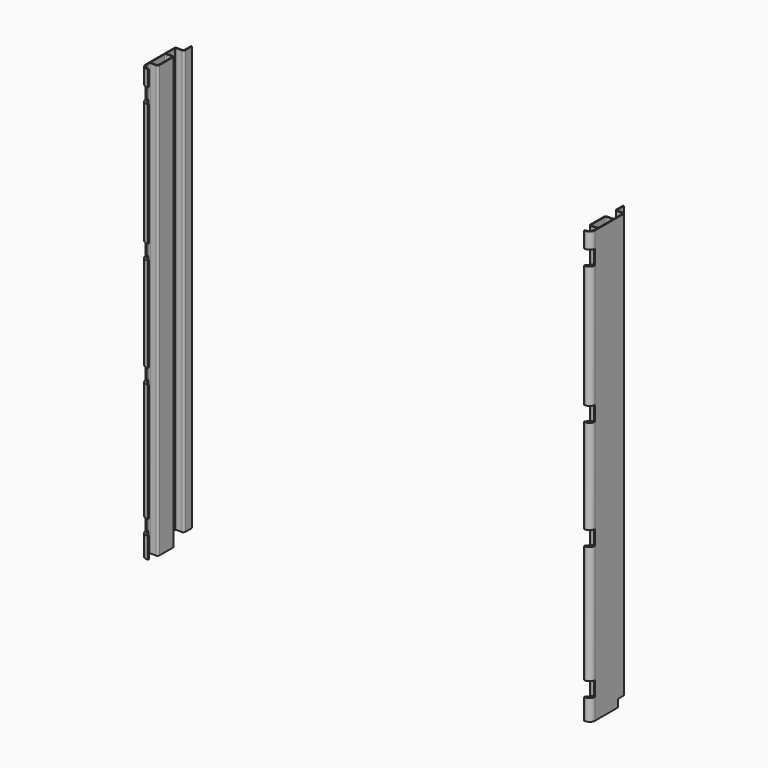
from build123d import *

# Parameters (mm, degrees)
F1_DEPTH  = 2337
F2_W      = 58.9122746438
F2_H      = 85
F2_W_2    = 42.5596956462
F2_W_3    = 40.1068006009
F2_W_4    = 37.0883546919
F2_H_2    = 41
F3_DEPTH  = 55
F5_DEPTH  = 2
F7_DEPTH  = 2
F9_DEPTH  = 2
F11_DEPTH = 2
F13_DEPTH = 2
F15_DEPTH = 2
F17_DEPTH = 2
F19_DEPTH = 2
F21_DEPTH = 2337


# Not quite as in the source:
# - a feature names something its author has since deleted; it is built from what else it names


with BuildPart() as f1:
    # F0 (on Top) → F1 (new body)
    with BuildSketch(Plane.XY):
        with BuildLine():
            Line((-45, 88.8779433221), (-45, 133.8779433221))
            Line((-45, 133.8779433221), (-50, 133.8779433221))
            Line((-50, 133.8779433221), (-50, 88.8779433221))
            ThreePointArc((-50, 88.8779433221), (-47.0710678119, 81.8068755102), (-40, 78.8779433221))
            Line((-40, 78.8779433221), (-10, 78.8779433221))
            ThreePointArc((-10, 78.8779433221), (-6.4644660941, 77.413477228), (-5, 73.8779433221))
            Line((-5, 73.8779433221), (-5, 19.8779433221))
            ThreePointArc((-5, 19.8779433221), (-6.4644660941, 16.3424094161), (-10, 14.8779433221))
            Line((-10, 14.8779433221), (-40, 14.8779433221))
            ThreePointArc((-40, 14.8779433221), (-47.0710678119, 11.9490111339), (-50, 4.8779433221))
            Line((-50, 4.8779433221), (-50, -86.1220566779))
            ThreePointArc((-50, -86.1220566779), (-47.0710678119, -93.1931244898), (-40, -96.1220566779))
            Line((-40, -96.1220566779), (-10, -96.1220566779))
            ThreePointArc((-10, -96.1220566779), (-6.4644660941, -97.586522772), (-5, -101.1220566779))
            Line((-5, -101.1220566779), (-5, -112.1220566779))
            ThreePointArc((-5, -112.1220566779), (-13.7867965644, -133.3352601135), (-35, -142.1220566779))
            Line((-35, -142.1220566779), (-37, -142.1220566779))
            Line((-37, -142.1220566779), (-37, -147.1220566779))
            Line((-37, -147.1220566779), (-30, -147.1220566779))
            ThreePointArc((-30, -147.1220566779), (-8.7867965644, -138.3352601135), (0, -117.1220566779))
            Line((0, -117.1220566779), (0, 73.8779433221))
            ThreePointArc((0, 73.8779433221), (-2.9289321881, 80.9490111339), (-10, 83.8779433221))
            Line((-10, 83.8779433221), (-40, 83.8779433221))
            ThreePointArc((-40, 83.8779433221), (-43.5355339059, 85.3424094161), (-45, 88.8779433221))
        make_face()
        with BuildLine():
            ThreePointArc((-45, 4.8779433221), (-43.5355339059, 8.413477228), (-40, 9.8779433221))
            Line((-40, 9.8779433221), (-10, 9.8779433221))
            ThreePointArc((-10, 9.8779433221), (-6.4644660941, 8.413477228), (-5, 4.8779433221))
            Line((-5, 4.8779433221), (-5, -86.1220566779))
            ThreePointArc((-5, -86.1220566779), (-6.4644660941, -89.6575905839), (-10, -91.1220566779))
            Line((-10, -91.1220566779), (-40, -91.1220566779))
            ThreePointArc((-40, -91.1220566779), (-43.5355339059, -89.6575905839), (-45, -86.1220566779))
            Line((-45, -86.1220566779), (-45, 4.8779433221))
        make_face(mode=Mode.SUBTRACT)
    extrude(amount=F1_DEPTH)

    # F2 (on face) → F3 (cut)
    with BuildSketch(Plane.YZ):
        Polygon((135.9497308731, 41), (73.8779433221, 41), (73.8779433221, 0), (36.7895886302, 0), (36.7895886302, -10.0573040545), (135.9497308731, -10.0573040545), align=None)
        with Locations((-146.5781939998, 153.5)):
            Rectangle(F2_W, F2_H)
        with Locations((-138.401904501, 873.5)):
            Rectangle(F2_W_2, F2_H)
        with Locations((-137.1754569784, 1465.5)):
            Rectangle(F2_W_3, F2_H)
        with Locations((-137.1754569784, 2210.5)):
            Rectangle(F2_W_3, F2_H)
        with Locations((55.3337659761, 20.5)):
            Rectangle(F2_W_4, F2_H_2)
    extrude(amount=-F3_DEPTH, mode=Mode.SUBTRACT)

    # F4 (on face) → F5 (join)
    with BuildSketch(Plane(origin=(0, 0, 2253), x_dir=(1, 0, 0), z_dir=(0, 0, -1))):
        with BuildLine():
            Line((-35, 142.1220566779), (-37, 142.1220566779))
            Line((-37, 142.1220566779), (0, 101.1220566779))
            Line((0, 101.1220566779), (0, 117.1220566779))
            Line((0, 117.1220566779), (-5.4196010845, 117.1220566779))
            ThreePointArc((-5.4196010845, 117.1220566779), (-15.635083269, 135.0349351527), (-35, 142.1220566779))
        make_face()
        with BuildLine():
            Line((-30, 147.1220566779), (-37, 147.1220566779))
            Line((-37, 147.1220566779), (-37, 142.1220566779))
            Line((-37, 142.1220566779), (-35, 142.1220566779))
            ThreePointArc((-35, 142.1220566779), (-15.635083269, 135.0349351527), (-5.4196010845, 117.1220566779))
            Line((-5.4196010845, 117.1220566779), (0, 117.1220566779))
            ThreePointArc((0, 117.1220566779), (-8.7867965644, 138.3352601135), (-30, 147.1220566779))
        make_face()
    extrude(amount=F5_DEPTH)

    # F6 (on face) → F7 (join)
    with BuildSketch(Plane.XY.offset(2168)):
        with BuildLine():
            Line((0, -101.1220566779), (-37, -142.1220566779))
            Line((-37, -142.1220566779), (-35, -142.1220566779))
            ThreePointArc((-35, -142.1220566779), (-15.635083269, -135.0349351527), (-5.4196010845, -117.1220566779))
            Line((-5.4196010845, -117.1220566779), (0, -117.1220566779))
            Line((0, -117.1220566779), (0, -101.1220566779))
        make_face()
        with BuildLine():
            Line((-37, -142.1220566779), (-37, -147.1220566779))
            Line((-37, -147.1220566779), (-30, -147.1220566779))
            ThreePointArc((-30, -147.1220566779), (-8.7867965644, -138.3352601135), (0, -117.1220566779))
            Line((0, -117.1220566779), (-5.4196010845, -117.1220566779))
            ThreePointArc((-5.4196010845, -117.1220566779), (-15.635083269, -135.0349351527), (-35, -142.1220566779))
            Line((-35, -142.1220566779), (-37, -142.1220566779))
        make_face()
    extrude(amount=F7_DEPTH)

    # F8 (on face) → F9 (join)
    with BuildSketch(Plane(origin=(0, 0, 1508), x_dir=(1, 0, 0), z_dir=(0, 0, -1))):
        with BuildLine():
            Line((-35, 142.1220566779), (-37, 142.1220566779))
            Line((-37, 142.1220566779), (0, 101.1220566779))
            Line((0, 101.1220566779), (0, 117.1220566779))
            Line((0, 117.1220566779), (-5.4196010845, 117.1220566779))
            ThreePointArc((-5.4196010845, 117.1220566779), (-15.635083269, 135.0349351527), (-35, 142.1220566779))
        make_face()
        with BuildLine():
            Line((-30, 147.1220566779), (-37, 147.1220566779))
            Line((-37, 147.1220566779), (-37, 142.1220566779))
            Line((-37, 142.1220566779), (-35, 142.1220566779))
            ThreePointArc((-35, 142.1220566779), (-15.635083269, 135.0349351527), (-5.4196010845, 117.1220566779))
            Line((-5.4196010845, 117.1220566779), (0, 117.1220566779))
            ThreePointArc((0, 117.1220566779), (-8.7867965644, 138.3352601135), (-30, 147.1220566779))
        make_face()
    extrude(amount=F9_DEPTH)

    # F10 (on face) → F11 (join)
    with BuildSketch(Plane.XY.offset(1423)):
        with BuildLine():
            Line((-35, -142.1220566779), (-37, -142.1220566779))
            Line((-37, -142.1220566779), (-37, -147.1220566779))
            Line((-37, -147.1220566779), (-30, -147.1220566779))
            ThreePointArc((-30, -147.1220566779), (-8.7867965644, -138.3352601135), (0, -117.1220566779))
            Line((0, -117.1220566779), (-5.4196010845, -117.1220566779))
            ThreePointArc((-5.4196010845, -117.1220566779), (-15.635083269, -135.0349351527), (-35, -142.1220566779))
        make_face()
        with BuildLine():
            Line((0, -101.1220566779), (-37, -142.1220566779))
            Line((-37, -142.1220566779), (-35, -142.1220566779))
            ThreePointArc((-35, -142.1220566779), (-15.635083269, -135.0349351527), (-5.4196010845, -117.1220566779))
            Line((-5.4196010845, -117.1220566779), (0, -117.1220566779))
            Line((0, -117.1220566779), (0, -101.1220566779))
        make_face()
    extrude(amount=F11_DEPTH)

    # F12 (on face) → F13 (join)
    with BuildSketch(Plane(origin=(0, 0, 916), x_dir=(1, 0, 0), z_dir=(0, 0, -1))):
        with BuildLine():
            Line((-35, 142.1220566779), (-37, 142.1220566779))
            Line((-37, 142.1220566779), (0, 101.1220566779))
            Line((0, 101.1220566779), (0, 117.1220566779))
            Line((0, 117.1220566779), (-5.4196010845, 117.1220566779))
            ThreePointArc((-5.4196010845, 117.1220566779), (-15.635083269, 135.0349351527), (-35, 142.1220566779))
        make_face()
        with BuildLine():
            Line((-37, 147.1220566779), (-37, 142.1220566779))
            Line((-37, 142.1220566779), (-35, 142.1220566779))
            ThreePointArc((-35, 142.1220566779), (-15.635083269, 135.0349351527), (-5.4196010845, 117.1220566779))
            Line((-5.4196010845, 117.1220566779), (0, 117.1220566779))
            ThreePointArc((0, 117.1220566779), (-8.7867965644, 138.3352601135), (-30, 147.1220566779))
            Line((-30, 147.1220566779), (-37, 147.1220566779))
        make_face()
    extrude(amount=F13_DEPTH)

    # F14 (on face) → F15 (join)
    with BuildSketch(Plane.XY.offset(831)):
        with BuildLine():
            Line((0, -101.1220566779), (-37, -142.1220566779))
            Line((-37, -142.1220566779), (-35, -142.1220566779))
            ThreePointArc((-35, -142.1220566779), (-15.635083269, -135.0349351527), (-5.4196010845, -117.1220566779))
            Line((-5.4196010845, -117.1220566779), (0, -117.1220566779))
            Line((0, -117.1220566779), (0, -101.1220566779))
        make_face()
        with BuildLine():
            Line((-35, -142.1220566779), (-37, -142.1220566779))
            Line((-37, -142.1220566779), (-37, -147.1220566779))
            Line((-37, -147.1220566779), (-30, -147.1220566779))
            ThreePointArc((-30, -147.1220566779), (-8.7867965644, -138.3352601135), (0, -117.1220566779))
            Line((0, -117.1220566779), (-5.4196010845, -117.1220566779))
            ThreePointArc((-5.4196010845, -117.1220566779), (-15.635083269, -135.0349351527), (-35, -142.1220566779))
        make_face()
    extrude(amount=F15_DEPTH)

    # F16 (on face) → F17 (join)
    with BuildSketch(Plane(origin=(0, 0, 196), x_dir=(1, 0, 0), z_dir=(0, 0, -1))):
        with BuildLine():
            Line((-35, 142.1220566779), (-37, 142.1220566779))
            Line((-37, 142.1220566779), (0, 101.1220566779))
            Line((0, 101.1220566779), (0, 117.1220566779))
            Line((0, 117.1220566779), (-5.4196010845, 117.1220566779))
            ThreePointArc((-5.4196010845, 117.1220566779), (-15.635083269, 135.0349351527), (-35, 142.1220566779))
        make_face()
        with BuildLine():
            Line((-37, 147.1220566779), (-37, 142.1220566779))
            Line((-37, 142.1220566779), (-35, 142.1220566779))
            ThreePointArc((-35, 142.1220566779), (-15.635083269, 135.0349351527), (-5.4196010845, 117.1220566779))
            Line((-5.4196010845, 117.1220566779), (0, 117.1220566779))
            ThreePointArc((0, 117.1220566779), (-8.7867965644, 138.3352601135), (-30, 147.1220566779))
            Line((-30, 147.1220566779), (-37, 147.1220566779))
        make_face()
    extrude(amount=F17_DEPTH)

    # F18 (on face) → F19 (join)
    with BuildSketch(Plane.XY.offset(111)):
        with BuildLine():
            Line((0, -101.1220566779), (-37, -142.1220566779))
            Line((-37, -142.1220566779), (-35, -142.1220566779))
            ThreePointArc((-35, -142.1220566779), (-15.635083269, -135.0349351527), (-5.4196010845, -117.1220566779))
            Line((-5.4196010845, -117.1220566779), (0, -117.1220566779))
            Line((0, -117.1220566779), (0, -101.1220566779))
        make_face()
        with BuildLine():
            Line((-35, -142.1220566779), (-37, -142.1220566779))
            Line((-37, -142.1220566779), (-37, -147.1220566779))
            Line((-37, -147.1220566779), (-30, -147.1220566779))
            ThreePointArc((-30, -147.1220566779), (-8.7867965644, -138.3352601135), (0, -117.1220566779))
            Line((0, -117.1220566779), (-5.4196010845, -117.1220566779))
            ThreePointArc((-5.4196010845, -117.1220566779), (-15.635083269, -135.0349351527), (-35, -142.1220566779))
        make_face()
    extrude(amount=F19_DEPTH)

    # F20 (on face) → F21 (cut)
    with BuildSketch(Plane(origin=(0, 0, 111), x_dir=(1, 0, 0), z_dir=(0, 0, -1))):
        with BuildLine():
            ThreePointArc((-13.8044904411, 130.8858355746), (-19.4539209941, 131.1755499619), (-19.7436353814, 125.5261194089))
            Line((-19.7436353814, 125.5261194089), (-13.8044904411, 130.8858355746))
        make_face()
        with BuildLine():
            Line((-13.8044904411, 130.8858355746), (-19.7436353814, 125.5261194089))
            ThreePointArc((-19.7436353814, 125.5261194089), (-15.3384950586, 124.4724610607), (-12.7740629113, 128.2059774917))
            ThreePointArc((-12.7740629113, 128.2059774917), (-13.0405464803, 129.6415453444), (-13.8044904411, 130.8858355746))
        make_face()
    extrude(amount=-F21_DEPTH, mode=Mode.SUBTRACT)


with BuildPart() as f23_1:
    # F23: instance of F1
    add(f1.part.mirror(Plane(origin=(-1217, -40.6220566779, 1168.5), x_dir=(0, -1, 0), z_dir=(-1, 0, 0))))


solid = Compound([f1.part, f23_1.part])
